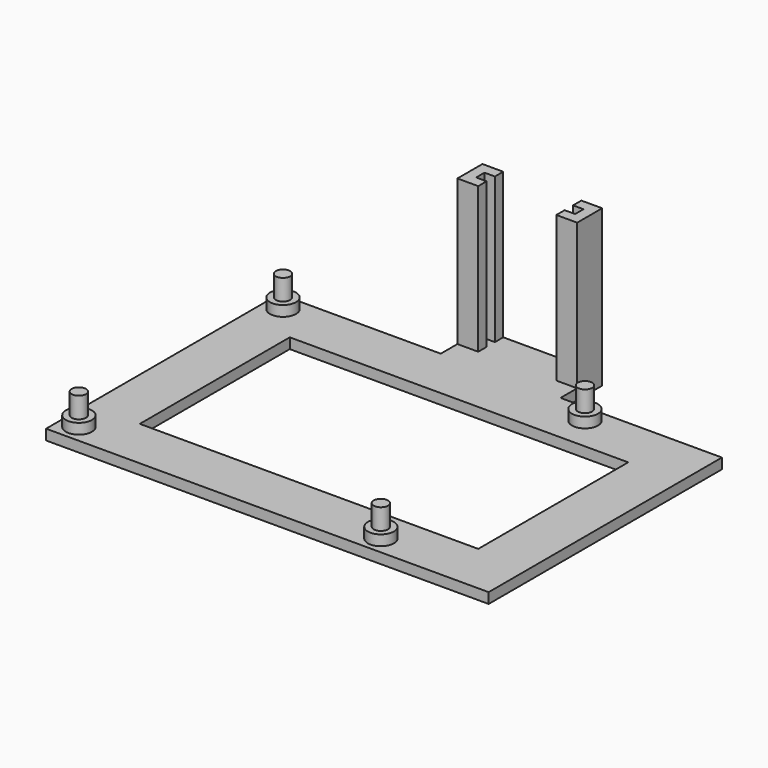
from build123d import *

# Parameters (mm, degrees)
F1_DEPTH = 30
F0_R     = 2.5
F0_R_2   = 1.375
F2_DEPTH = 4
F3_DEPTH = 8
F0_W     = 65
F0_H     = 36
F4_DEPTH = 2


with BuildPart() as f1:
    # F0 (on Top) → F1 (new body)
    with BuildSketch(Plane.XY):
        Polygon((31, 66), (31, 60), (35, 60), (35, 62), (33, 62), (33, 64), (35, 64), (35, 66), align=None)
    extrude(amount=F1_DEPTH)



with BuildPart() as f1b:
    # F0 (on Top) → F1, piece 2 (new body)
    with BuildSketch(Plane.XY):
        Polygon((50, 60), (54, 60), (54, 66), (50, 66), (50, 64), (52, 64), (52, 62), (50, 62), align=None)
    extrude(amount=F1_DEPTH)


with BuildPart() as f2:
    # F0 (on Top) → F2 (new body)
    with BuildSketch(Plane.XY):
        with Locations((3.5, 52.5)):
            Circle(F0_R)
        with Locations((3.5, 52.5)):
            Circle(F0_R_2, mode=Mode.SUBTRACT)
    extrude(amount=F2_DEPTH)

    # F0 (on Top) → F3 (join)
    with BuildSketch(Plane.XY):
        with Locations((3.5, 52.5)):
            Circle(F0_R_2)
    extrude(amount=F3_DEPTH)


with BuildPart() as f2b:
    # F0 (on Top) → F2, piece 2 (new body)
    with BuildSketch(Plane.XY):
        with Locations((61.5, 52.5)):
            Circle(F0_R)
        with Locations((61.5, 52.5)):
            Circle(F0_R_2, mode=Mode.SUBTRACT)
    extrude(amount=F2_DEPTH)

    # F0 (on Top) → F3, piece 2 (join)
    with BuildSketch(Plane.XY):
        with Locations((61.5, 52.5)):
            Circle(F0_R_2)
    extrude(amount=F3_DEPTH)


with BuildPart() as f2c:
    # F0 (on Top) → F2, piece 3 (new body)
    with BuildSketch(Plane.XY):
        with Locations((61.5, 3.5)):
            Circle(F0_R)
        with Locations((61.5, 3.5)):
            Circle(F0_R_2, mode=Mode.SUBTRACT)
    extrude(amount=F2_DEPTH)

    # F0 (on Top) → F3, piece 3 (join)
    with BuildSketch(Plane.XY):
        with Locations((61.5, 3.5)):
            Circle(F0_R_2)
    extrude(amount=F3_DEPTH)


with BuildPart() as f2d:
    # F0 (on Top) → F2, piece 4 (new body)
    with BuildSketch(Plane.XY):
        with Locations((3.5, 3.5)):
            Circle(F0_R)
        with Locations((3.5, 3.5)):
            Circle(F0_R_2, mode=Mode.SUBTRACT)
    extrude(amount=F2_DEPTH)

    # F0 (on Top) → F3, piece 4 (join)
    with BuildSketch(Plane.XY):
        with Locations((3.5, 3.5)):
            Circle(F0_R_2)
    extrude(amount=F3_DEPTH)


with BuildPart() as f1_1:
    add(f1.part)

    add(f1b.part)  # F4 merges F1b

    add(f2.part)  # F4 merges F2

    add(f2b.part)  # F4 merges F2b

    add(f2c.part)  # F4 merges F2c

    add(f2d.part)  # F4 merges F2d
    # F0 (on Top) → F4 (join)
    with BuildSketch(Plane.XY):
        Polygon((0, 28), (0, 0), (85, 0), (85, 28), (85, 56), (54, 56), (54, 60), (50, 60), (50, 62), (52, 62), (52, 64), (50, 64), (50, 66), (35, 66), (35, 64), (33, 64), (33, 62), (35, 62), (35, 60), (31, 60), (31, 56), (0, 56), align=None)
        with Locations((3.5, 3.5)):
            Circle(F0_R, mode=Mode.SUBTRACT)
        with Locations((61.5, 3.5)):
            Circle(F0_R, mode=Mode.SUBTRACT)
        with Locations((42.5, 28)):
            Rectangle(F0_W, F0_H, mode=Mode.SUBTRACT)
        with Locations((3.5, 52.5)):
            Circle(F0_R, mode=Mode.SUBTRACT)
        with Locations((61.5, 52.5)):
            Circle(F0_R, mode=Mode.SUBTRACT)
    extrude(amount=F4_DEPTH)


solid = f1_1.part
